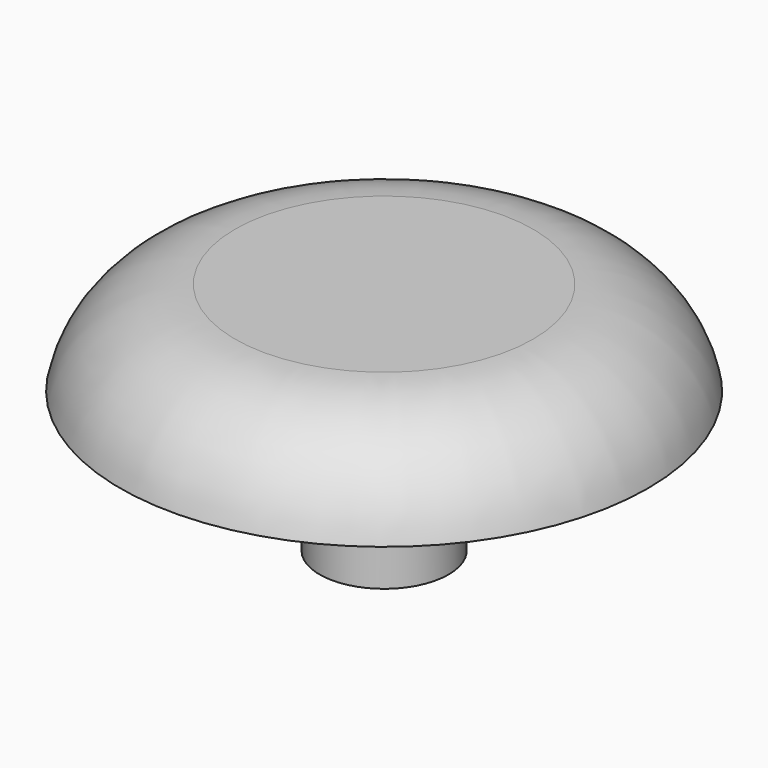
from build123d import *

# Parameters (mm, degrees)
F0_R     = 2.75
F1_DEPTH = 6
F2_R     = 11.25
F3_DEPTH = 4


# Not quite as in the source:
# - a fillet or chamfer that OpenCascade refuses, or shapes differently, is made with other operations: its cross-section is extruded or revolved along the edge and cut away or added


with BuildPart() as f1:
    # F0 (on Top) → F1 (new body)
    with BuildSketch(Plane.XY):
        Circle(F0_R)
    extrude(amount=F1_DEPTH)

    # F2 (on face) → F3 (join)
    with BuildSketch(Plane.XY.offset(6)):
        Circle(F2_R)
    extrude(amount=F3_DEPTH)

    # F4: fillet of radius 5 on 1 edges, made by hand

    # F4_s1 → F4_t2 (revolve, cut)
    with BuildSketch(Plane.XZ):
        with BuildLine():
            ThreePointArc((11.25, 6), (9.5132981746, 8.8729833462), (6.3510205144, 10))
            Line((6.3510205144, 10), (11.25, 10))
            Line((11.25, 10), (11.25, 6))
        make_face()
    revolve(axis=Axis((0, 0, 10), (0, 0, 1)), mode=Mode.SUBTRACT)


solid = f1.part
